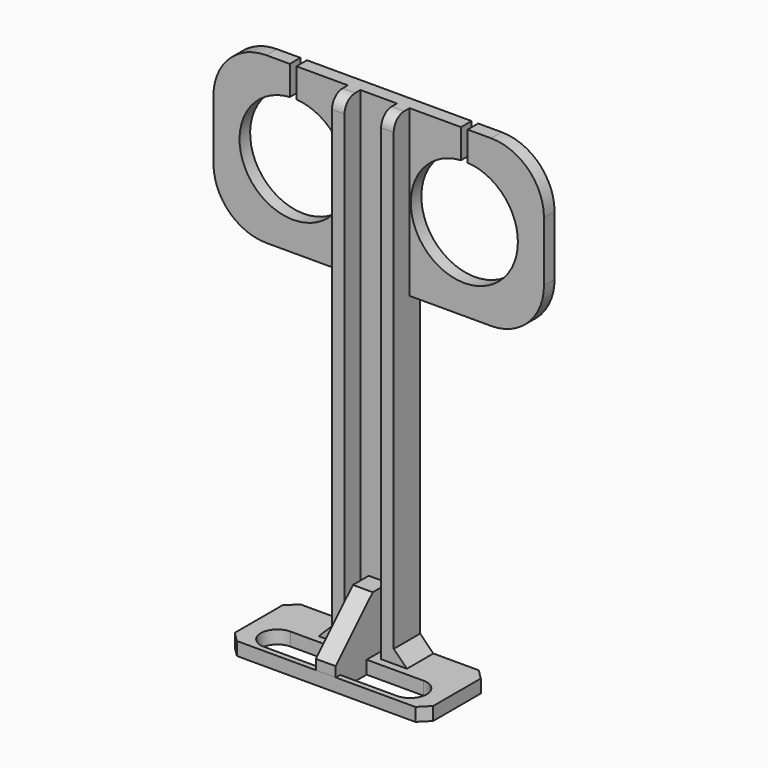
from build123d import *
from build123d import SkipClean  # not in build123d's __all__

# Parameters (mm, degrees)
F1_DEPTH      = 2
F0_W          = 5.54
F0_H          = 25
F0_W_2        = 1.9
F0_W_3        = 2.5
F0_H_2        = 2.5
F2_DEPTH      = 5
F3_DEPTH      = 5
F4_DEPTH      = 7
F5_SIZE       = 7
F8_DEPTH      = 2
F9_SIZE       = 1.5
F10_SIZE      = 1.5
F11_SIZE      = 1.5
F12_R         = 8
F13_R         = 2
F14_T4_DEPTH  = 20.4300979278
F14_T10_DEPTH = 20.4300979278


# Not quite as in the source:
# - a fillet or chamfer that OpenCascade refuses, or shapes differently, is made with other operations: its cross-section is extruded or revolved along the edge and cut away or added
# - ends of sketch curves that miss each other by under 0.0002 mm in the source are joined
# - a feature names something its author has since deleted; it is built from what else it names


with BuildPart() as f1:
    # F0 (on Front) → F1 (new body)
    with BuildSketch(Plane.XZ):
        with BuildLine():
            Line((-25, 38.2831491688), (-4.67, 38.2831491688))
            Line((-4.67, 38.2831491688), (-4.67, 63.2831491688))
            Line((-4.67, 63.2831491688), (-12.45, 63.2831491688))
            Line((-12.45, 63.2831491688), (-12.45, 58.8677023414))
            ThreePointArc((-12.45, 58.8677023414), (-7.0483053281, 56.3311217715), (-4.85, 50.7831491688))
            ThreePointArc((-4.85, 50.7831491688), (-18.4979726027, 44.8814544969), (-13.45, 58.8677023414))
            Line((-13.45, 58.8677023414), (-13.45, 63.2831491688))
            Line((-13.45, 63.2831491688), (-25, 63.2831491688))
            Line((-25, 63.2831491688), (-25, 38.2831491688))
        make_face()
    extrude(amount=F1_DEPTH)



with BuildPart() as f1b:
    # F0 (on Front) → F1, piece 2 (new body)
    with BuildSketch(Plane.XZ):
        with BuildLine():
            Line((4.67, 38.2831491688), (25, 38.2831491688))
            Line((25, 38.2831491688), (25, 63.2831491688))
            Line((25, 63.2831491688), (13.45, 63.2831491688))
            Line((13.45, 63.2831491688), (13.45, 58.8677023414))
            ThreePointArc((13.45, 58.8677023414), (18.8516946719, 56.3311217715), (21.05, 50.7831491688))
            ThreePointArc((21.05, 50.7831491688), (7.4020273973, 44.8814544969), (12.45, 58.8677023414))
            Line((12.45, 58.8677023414), (12.45, 63.2831491688))
            Line((12.45, 63.2831491688), (4.67, 63.2831491688))
            Line((4.67, 63.2831491688), (4.67, 38.2831491688))
        make_face()
    extrude(amount=F1_DEPTH)


with BuildPart() as f1c:
    # F0 (on Front) → F1, piece 3 (new body)
    with BuildSketch(Plane.XZ):
        with Locations((0, 50.7831491688)):
            Rectangle(F0_W, F0_H)
        Polygon((2.77, -9.5068508312), (2.77, 38.2831491688), (-2.77, 38.2831491688), (-2.77, -9.5068508312), (-1.5, -9.5068508312), (-1.5, -0.9968508312), (1.5, -0.9968508312), (1.5, -9.5068508312), align=None)
    extrude(amount=F1_DEPTH)


with BuildPart() as f1_1:
    add(f1.part, clean=False)

    add(f1b.part)  # F2 merges F1b

    add(f1c.part)  # F2 merges F1c
    # F0 (on Front) → F2 (join)
    with BuildSketch(Plane.XZ):
        Polygon((-2.77, -9.5068508312), (-2.77, 38.2831491688), (-4.67, 38.2831491688), (-4.67, 0), (-4.67, -7.0068508312), (-4.67, -9.5068508312), align=None)
        Polygon((4.67, -7.0068508312), (4.67, 38.2831491688), (2.77, 38.2831491688), (2.77, -9.5068508312), (4.67, -9.5068508312), align=None)
        with Locations((3.72, 50.7831491688)):
            Rectangle(F0_W_2, F0_H)
        with Locations((-3.72, 50.7831491688)):
            Rectangle(F0_W_2, F0_H)
        with Locations((-5.92, -8.2568508312)):
            Rectangle(F0_W_3, F0_H_2)
        with Locations((5.92, -8.2568508312)):
            Rectangle(F0_W_3, F0_H_2)
    extrude(amount=F2_DEPTH)

    # F0 (on Front) → F3 (join)
    with BuildSketch(Plane.XZ):
        Polygon((1.5, -11.5068508312), (1.5, -9.5068508312), (1.5, -0.9968508312), (-1.5, -0.9968508312), (-1.5, -9.5068508312), (-1.5, -11.5068508312), align=None)
    extrude(amount=F3_DEPTH)

    # F4 (add): a face of the model
    f4_faces = [f1_1.faces().sort_by_distance(p)[0] for p in [
        (0, -5, -6.2518508312),
    ]]
    extrude(f4_faces, amount=F4_DEPTH)

    # F5
    f5_edges = [f1_1.edges().sort_by_distance(p)[0] for p in [
        (0, -12, -0.996851),
    ]]
    chamfer(f5_edges, length=F5_SIZE)

    # F7 (on face) → F8 (join)
    with BuildSketch(Plane(origin=(0, 0, -9.5068508312), x_dir=(1, 0, 0), z_dir=(0, 0, -1))):
        Polygon((15.0385206658, 12.000000352), (0.0385206658, 12.000000352), (-14.9614793342, 12.000000352), (-14.9614793342, 3.52e-07), (1.5, 3.52e-07), (1.5, 2), (2.77, 2), (2.77, 5), (7.17, 5), (7.17, 0), (15.0385206658, 3.52e-07), align=None)
        with BuildLine():
            ThreePointArc((-10.0064205471, 6.1577448677), (-12.5064205471, 8.6577448677), (-10.0064205471, 11.1577448677))
            Line((-10.0064205471, 11.1577448677), (10.0834618788, 11.1577448677))
            ThreePointArc((10.0834618788, 11.1577448677), (11.8512288318, 10.4255118207), (12.5834618788, 8.6577448677))
            ThreePointArc((12.5834618788, 8.6577448677), (11.8512288318, 6.8899779148), (10.0834618788, 6.1577448677))
            Line((10.0834618788, 6.1577448677), (-10.0064205471, 6.1577448677))
        make_face(mode=Mode.SUBTRACT)
        Polygon((1.5, 2), (1.5, 0), (7.17, 3.52e-07), (7.17, 5), (2.77, 5), (2.77, 2), align=None)
    with SkipClean():  # cleaning this boolean's faces spoils the solid; the shape is the same uncleaned
        extrude(amount=F8_DEPTH)

    # F9
    f9_edges = [f1_1.edges().sort_by_distance(p)[0] for p in [
        (15.038521, -12, -10.506851),
    ]]
    chamfer(f9_edges, length=F9_SIZE)

    # F10
    f10_edges = [f1_1.edges().sort_by_distance(p)[0] for p in [
        (-14.961479, -12, -10.506851),
    ]]
    chamfer(f10_edges, length=F10_SIZE)

    # F11
    f11_edges = [f1_1.edges().sort_by_distance(p)[0] for p in [
        (-14.961479, 0, -10.506851),
        (15.038521, 0, -10.506851),
    ]]
    chamfer(f11_edges, length=F11_SIZE)

    # F12
    f12_edges = [f1_1.edges().sort_by_distance(p)[0] for p in [
        (25, -1, 38.283149),
        (-25, -1, 38.283149),
        (-25, -1, 63.283149),
        (25, -1, 63.283149),
    ]]
    fillet(f12_edges, radius=F12_R)

    # F13
    f13_edges = [f1_1.edges().sort_by_distance(p)[0] for p in [
        (3.72, -5, 63.283149),
        (-3.72, -5, 63.283149),
    ]]
    fillet(f13_edges, radius=F13_R)

    # F14: chamfer of 3 on 2 edges, made by hand


with BuildPart() as f14_tool2:
    # F14_s3 → F14_t4 (new body)
    with BuildSketch(Plane.XZ.offset(-7.7150489639)):
        Polygon((4.17, -7.0068508312), (7.17, -10.0068508312), (7.17, -7.0068508312), align=None)
    extrude(amount=F14_T4_DEPTH)

    split(bisect_by=Plane.YZ.offset(4.67), keep=Keep.TOP)

    split(bisect_by=Plane.XY.offset(-9.5068508312), keep=Keep.TOP)


with BuildPart() as f1_2:
    add(f1_1.part, clean=False)

    # F14_t1: cut F14_tool2
    add(f14_tool2.part, mode=Mode.SUBTRACT)


with BuildPart() as f14_tool8:
    # F14_s9 → F14_t10 (new body)
    with BuildSketch(Plane.XZ.offset(-7.7150489639)):
        Polygon((-7.17, -10.0068508312), (-4.17, -7.0068508312), (-7.17, -7.0068508312), align=None)
    extrude(amount=F14_T10_DEPTH)

    split(bisect_by=Plane.YZ.offset(-4.67), keep=Keep.BOTTOM)

    split(bisect_by=Plane.XY.offset(-9.5068508312), keep=Keep.TOP)


with BuildPart() as f1_3:
    add(f1_2.part, clean=False)

    # F14_t7: cut F14_tool8
    add(f14_tool8.part, mode=Mode.SUBTRACT)


solid = f1_3.part
